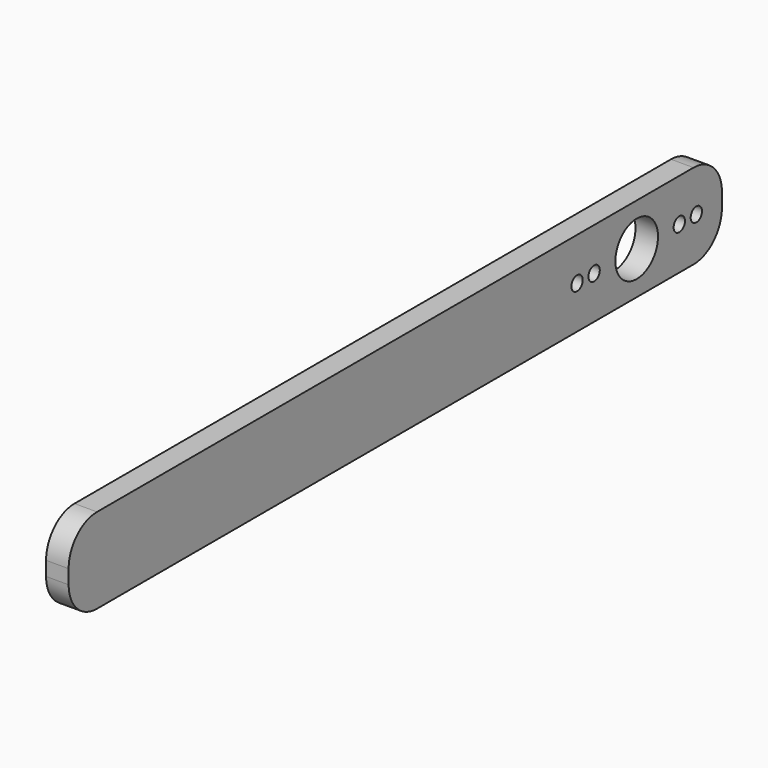
from build123d import *

# Parameters (mm, degrees)
F0_W     = 115
F0_H     = 12
F0_R     = 1
F0_R_2   = 3.75
F1_DEPTH = 3.175
F2_R     = 5
F3_R     = 5
F4_R     = 5
F5_R     = 5


# Not quite as in the source:
# - a length typed as a fraction of an inch, garbled in the dataset ("3 / 203.2 mm" for 3/8 in), is restored


with BuildPart() as f1:
    # F0 (on Right) → F1 (new body)
    with BuildSketch(Plane.YZ):
        with Locations((-42.5, 0)):
            Rectangle(F0_W, F0_H)
        with Locations((-10.5, 0)):
            Circle(F0_R, mode=Mode.SUBTRACT)
        with Locations((-7.5, 0)):
            Circle(F0_R, mode=Mode.SUBTRACT)
        Circle(F0_R_2, mode=Mode.SUBTRACT)
        with Locations((7.5, 0)):
            Circle(F0_R, mode=Mode.SUBTRACT)
        with Locations((10.5, 0)):
            Circle(F0_R, mode=Mode.SUBTRACT)
    extrude(amount=F1_DEPTH)

    # F2
    f2_edges = [f1.edges().sort_by_distance(p)[0] for p in [
        (1.5875, -100, 6),
    ]]
    fillet(f2_edges, radius=F2_R)

    # F3
    f3_edges = [f1.edges().sort_by_distance(p)[0] for p in [
        (1.5875, -100, -6),
    ]]
    fillet(f3_edges, radius=F3_R)

    # F4
    f4_edges = [f1.edges().sort_by_distance(p)[0] for p in [
        (1.5875, 15, 6),
    ]]
    fillet(f4_edges, radius=F4_R)

    # F5
    f5_edges = [f1.edges().sort_by_distance(p)[0] for p in [
        (1.5875, 15, -6),
    ]]
    fillet(f5_edges, radius=F5_R)


solid = f1.part
